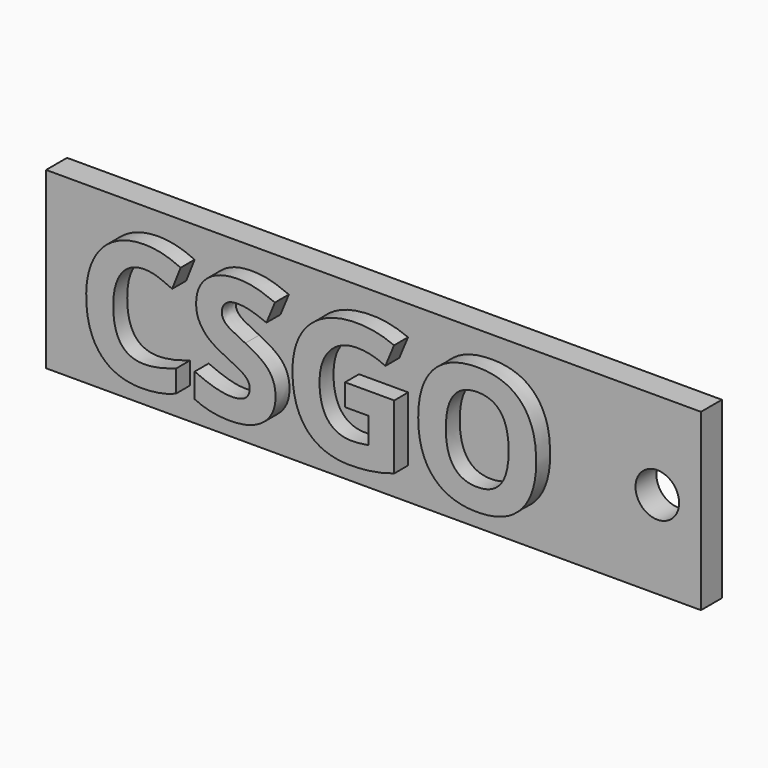
from build123d import *

# Parameters (mm, degrees)
F0_W         = 75
F0_H         = 20
F0_R         = 2.5
F1_DEPTH     = 3
F2_TEXT_SIZE = 19.8863647206
F3_DEPTH     = 2


# Not quite as in the source:
# - Text() gives the source's letters only with a copy of the font that has no kerning and outlines rounded to 1/6400 em; it was checked with that copy


with BuildPart() as f1:
    # F0 (on Front) → F1 (new body)
    with BuildSketch(Plane.XZ):
        with Locations((37.5, -10)):
            Rectangle(F0_W, F0_H)
        with Locations((70, -10)):
            Circle(F0_R, mode=Mode.SUBTRACT)
    extrude(amount=F1_DEPTH)

    # F2 (on face) → F3 (join)
    with BuildSketch(Plane.XZ.offset(3)):
        with Locations((5.0389645621, -16.9165129773)):
            Text('CSGO', F2_TEXT_SIZE, font='Open Sans', font_style=FontStyle.BOLD, text_align=(TextAlign.LEFT, TextAlign.BOTTOM))
    extrude(amount=F3_DEPTH)


solid = f1.part
